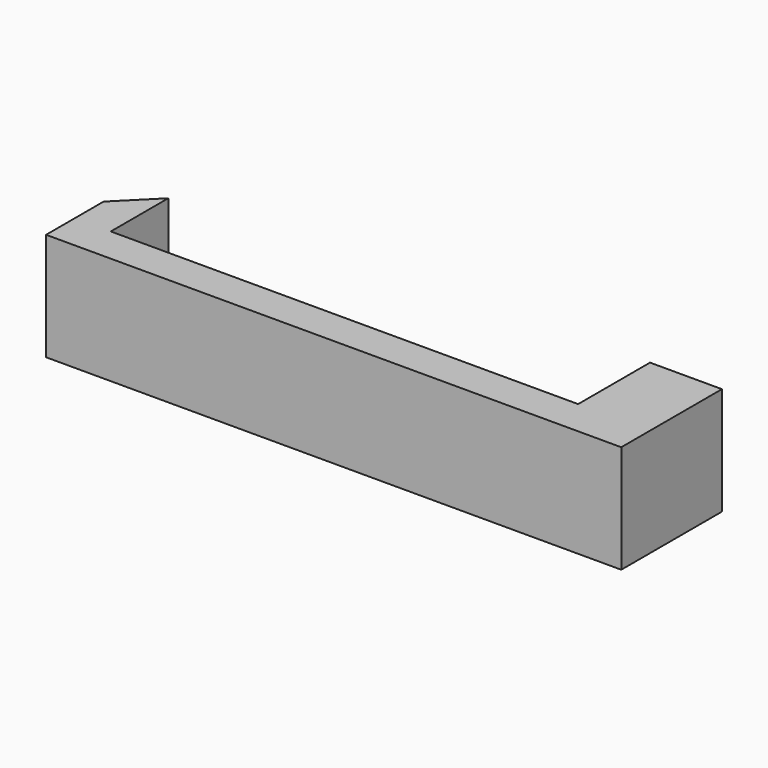
from build123d import *

# Parameters (mm, degrees)
F1_DEPTH = 6
F2_SIZE  = 1.99999


# Not quite as in the source:
# - a fillet or chamfer is up to 0.001 mm smaller than in the source, because OpenCascade refuses the exact size


with BuildPart() as f1:
    # F0 (on Top) → F1 (new body)
    with BuildSketch(Plane.XY):
        Polygon((-4, 7), (-4, 2), (-30, 2), (-30, 6), (-32, 6), (-32, 0), (0, 0), (0, 7), align=None)
    extrude(amount=F1_DEPTH)

    # F2 (size 2 in the source; OpenCascade refuses exactly that, so slightly less here)
    f2_edges = [f1.edges().sort_by_distance(p)[0] for p in [
        (-32, 6, 3),
    ]]
    chamfer(f2_edges, length=F2_SIZE)


solid = f1.part
